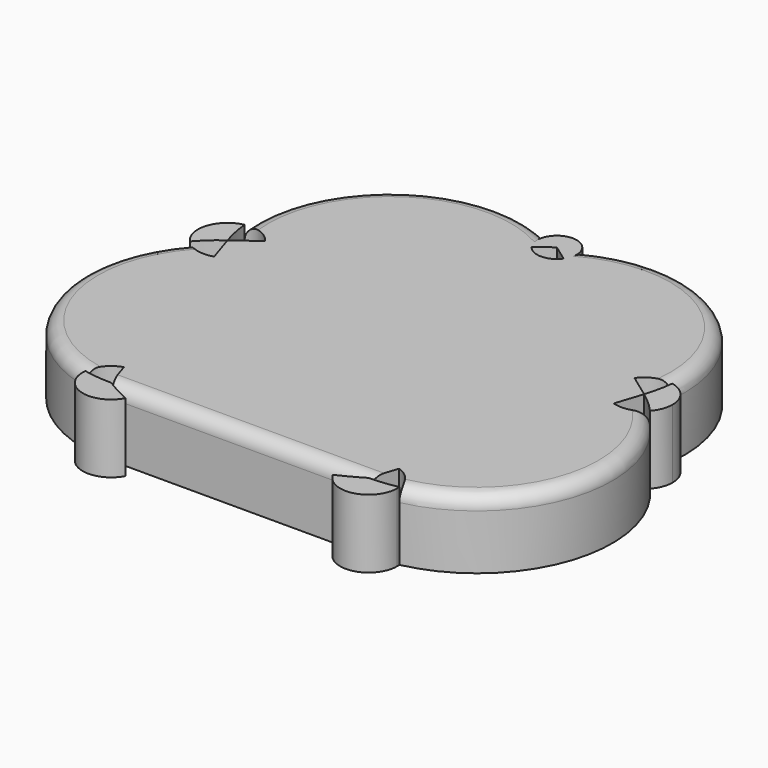
from build123d import *

# Parameters (mm, degrees)
F1_DEPTH     = 25.4
F2_T1_DEPTH  = 105.5253390088
F2_T6_ANGLE  = 135.1802111387
F2_S7_R      = 7.3377134681
F2_T8_DEPTH  = 54
F2_T10_ANGLE = 131.5087282243
F2_T12_ANGLE = 131.0798159324
F2_T16_ANGLE = 134.7112563381
F2_S17_R     = 7.3377134681
F2_T18_DEPTH = 54


# Not quite as in the source:
# - a fillet or chamfer that OpenCascade refuses, or shapes differently, is made with other operations: its cross-section is extruded or revolved along the edge and cut away or added


with BuildPart() as f1:
    # F0 (on Top) → F1 (new body)
    with BuildSketch(Plane.XY):
        with BuildLine():
            ThreePointArc((6.2360330355, 84.9896339964), (0, 88.4603161847), (-6.2360330355, 84.9896339964))
            ThreePointArc((-6.2360330355, 84.9896339964), (-3.047176806, 83.1703555454), (0, 81.1226027166))
            ThreePointArc((0, 81.1226027166), (3.047176806, 83.1703555454), (6.2360330355, 84.9896339964))
        make_face()
        with BuildLine():
            ThreePointArc((-58.1271279807, -64.5296013791), (-55.8437372027, -59.0194503726), (-50.9280340543, -55.6413591785))
            Line((-50.9280340543, -55.6413591785), (-73.7747197353, 14.6735092211))
            ThreePointArc((-73.7747197353, 14.6735092211), (-79.9572494224, 14.504659036), (-85.2415562442, 17.7184239823))
            ThreePointArc((-85.2415562442, 17.7184239823), (-95.2984726264, -31.1903792148), (-58.1271279807, -64.5296013791))
        make_face()
        with BuildLine():
            ThreePointArc((-6.2360330355, 84.9896339964), (-57.4611379356, 82.1562530019), (-79.3764959392, 35.7692235276))
            ThreePointArc((-79.3764959392, 35.7692235276), (-73.2123982771, 35.2631763666), (-68.3098743407, 31.4925739254))
            Line((-68.3098743407, 31.4925739254), (-5.9363348955, 76.8096029546))
            ThreePointArc((-5.9363348955, 76.8096029546), (-7.3327936166, 80.8539454711), (-6.2360330355, 84.9896339964))
        make_face()
        with BuildLine():
            ThreePointArc((0, 81.1226027166), (-3.047176806, 83.1703555454), (-6.2360330355, 84.9896339964))
            ThreePointArc((-6.2360330355, 84.9896339964), (-7.3327936166, 80.8539454711), (-5.9363348955, 76.8096029546))
            Line((-5.9363348955, 76.8096029546), (0, 81.1226027166))
        make_face()
        with BuildLine():
            Line((0, 81.1226027166), (5.9363348955, 76.8096029546))
            ThreePointArc((5.9363348955, 76.8096029546), (6.9785802085, 78.8551245551), (7.3377134681, 81.1226027166))
            ThreePointArc((7.3377134681, 81.1226027166), (7.0569208063, 83.1330523364), (6.2360330355, 84.9896339964))
            ThreePointArc((6.2360330355, 84.9896339964), (3.047176806, 83.1703555454), (0, 81.1226027166))
        make_face()
        with BuildLine():
            Line((5.9363348955, 76.8096029546), (68.6399088663, 31.2527898068))
            ThreePointArc((68.6399088663, 31.2527898068), (73.3795359036, 34.8903954871), (79.3356085511, 35.3609676448))
            ThreePointArc((79.3356085511, 35.3609676448), (57.631102228, 82.041368379), (6.2360330355, 84.9896339964))
            ThreePointArc((6.2360330355, 84.9896339964), (7.0569208063, 83.1330523364), (7.3377134681, 81.1226027166))
            ThreePointArc((7.3377134681, 81.1226027166), (6.9785802085, 78.8551245551), (5.9363348955, 76.8096029546))
        make_face()
        with BuildLine():
            Line((73.9007817067, 15.061488075), (50.9387999635, -55.6082251168))
            ThreePointArc((50.9387999635, -55.6082251168), (55.8696514193, -58.9960922671), (58.1613893706, -64.5222914193))
            ThreePointArc((58.1613893706, -64.5222914193), (95.3677177171, -30.9787541574), (84.9685108653, 18.0246769258))
            ThreePointArc((84.9685108653, 18.0246769258), (79.8733514993, 14.9044861347), (73.9007817067, 15.061488075))
        make_face()
        with BuildLine():
            ThreePointArc((-50.9280340543, -55.6413591785), (-41.5096192986, -57.1330895283), (-37.1804492093, -65.6295642257))
            Line((-37.1804492093, -65.6295642257), (37.1456099952, -65.6295642257))
            ThreePointArc((37.1456099952, -65.6295642257), (41.4891413224, -57.104904012), (50.9387999635, -55.6082251168))
            Line((50.9387999635, -55.6082251168), (73.9007817067, 15.061488075))
            ThreePointArc((73.9007817067, 15.061488075), (67.1454051401, 21.8168646416), (68.6399088663, 31.2527898068))
            Line((68.6399088663, 31.2527898068), (5.9363348955, 76.8096029546))
            ThreePointArc((5.9363348955, 76.8096029546), (0, 73.7848892486), (-5.9363348955, 76.8096029546))
            Line((-5.9363348955, 76.8096029546), (-68.3098743407, 31.4925739254))
            ThreePointArc((-68.3098743407, 31.4925739254), (-66.7574262862, 28.4457230645), (-66.2224891432, 25.0682628674))
            ThreePointArc((-66.2224891432, 25.0682628674), (-68.3098743407, 18.6439518093), (-73.7747197353, 14.6735092211))
            Line((-73.7747197353, 14.6735092211), (-50.9280340543, -55.6413591785))
        make_face()
        with BuildLine():
            ThreePointArc((68.6399088663, 31.2527898068), (67.1454051401, 21.8168646416), (73.9007817067, 15.061488075))
            Line((73.9007817067, 15.061488075), (77.1521799325, 25.0682628674))
            Line((77.1521799325, 25.0682628674), (68.6399088663, 31.2527898068))
        make_face()
        with BuildLine():
            Line((-77.1521799325, 25.0682628674), (-73.7747197353, 14.6735092211))
            ThreePointArc((-73.7747197353, 14.6735092211), (-68.3098743407, 18.6439518093), (-66.2224891432, 25.0682628674))
            ThreePointArc((-66.2224891432, 25.0682628674), (-66.7574262862, 28.4457230645), (-68.3098743407, 31.4925739254))
            Line((-68.3098743407, 31.4925739254), (-77.1521799325, 25.0682628674))
        make_face()
        with BuildLine():
            ThreePointArc((50.9387999635, -55.6082251168), (41.4891413224, -57.104904012), (37.1456099952, -65.6295642257))
            Line((37.1456099952, -65.6295642257), (47.6826695044, -65.6295642257))
            Line((47.6826695044, -65.6295642257), (50.9387999635, -55.6082251168))
        make_face()
        with BuildLine():
            Line((-47.6826695044, -65.6295642257), (-37.1804492093, -65.6295642257))
            ThreePointArc((-37.1804492093, -65.6295642257), (-41.5096192986, -57.1330895283), (-50.9280340543, -55.6413591785))
            Line((-50.9280340543, -55.6413591785), (-47.6826695044, -65.6295642257))
        make_face()
    extrude(amount=F1_DEPTH)

    # F2: fillet of radius 5.08 on 5 edges, made by hand

    # F2_s2 → F2_t1 (cut)
    with BuildSketch(Plane.YZ.offset(-52.7626695044)):
        with BuildLine():
            ThreePointArc((-65.6295642257, 20.32), (-64.1416666741, 23.9121024484), (-60.5495642257, 25.4))
            Line((-60.5495642257, 25.4), (-60.5495642257, 25.5016))
            Line((-60.5495642257, 25.5016), (-65.7311642257, 25.5016))
            Line((-65.7311642257, 25.5016), (-65.7311642257, 20.32))
            Line((-65.7311642257, 20.32), (-65.6295642257, 20.32))
        make_face()
    extrude(amount=F2_T1_DEPTH, mode=Mode.SUBTRACT)


with BuildPart() as f1b:
    # F0 (on Top) → F1, piece 2 (new body)
    with BuildSketch(Plane.XY):
        with BuildLine():
            ThreePointArc((77.1521799325, 25.0682628674), (81.2456293537, 21.7520811746), (84.9685108653, 18.0246769258))
            ThreePointArc((84.9685108653, 18.0246769258), (86.9743125522, 21.2956188385), (87.6739256131, 25.0682628674))
            ThreePointArc((87.6739256131, 25.0682628674), (85.3277720457, 31.6914664552), (79.3356085511, 35.3609676448))
            ThreePointArc((79.3356085511, 35.3609676448), (78.514647387, 30.157179414), (77.1521799325, 25.0682628674))
        make_face()
    extrude(amount=F1_DEPTH)


with BuildPart() as f1c:
    # F0 (on Top) → F1, piece 3 (new body)
    with BuildSketch(Plane.XY):
        with BuildLine():
            ThreePointArc((58.1613893706, -64.5222914193), (52.951199259, -65.3519775789), (47.6826695044, -65.6295642257))
            ThreePointArc((47.6826695044, -65.6295642257), (43.1052780453, -68.2425867862), (38.3851745007, -70.5880125472))
            ThreePointArc((38.3851745007, -70.5880125472), (50.2381895063, -75.8520365597), (58.2197290136, -65.6295642257))
            ThreePointArc((58.2197290136, -65.6295642257), (58.205133995, -65.0751599099), (58.1613893706, -64.5222914193))
        make_face()
    extrude(amount=F1_DEPTH)


with BuildPart() as f1d:
    # F0 (on Top) → F1, piece 4 (new body)
    with BuildSketch(Plane.XY):
        with BuildLine():
            ThreePointArc((-38.4168568148, -70.573383228), (-43.1206730546, -68.2343745884), (-47.6826695044, -65.6295642257))
            ThreePointArc((-47.6826695044, -65.6295642257), (-52.933779652, -65.3538152094), (-58.1271279807, -64.5296013791))
            ThreePointArc((-58.1271279807, -64.5296013791), (-50.7614884715, -75.6703562709), (-38.4168568148, -70.573383228))
        make_face()
    extrude(amount=F1_DEPTH)


with BuildPart() as f1e:
    # F0 (on Top) → F1, piece 5 (new body)
    with BuildSketch(Plane.XY):
        with BuildLine():
            ThreePointArc((-79.3764959392, 35.7692235276), (-87.5469335787, 28.4457230645), (-85.2415562442, 17.7184239823))
            ThreePointArc((-85.2415562442, 17.7184239823), (-81.3977483213, 21.614436135), (-77.1521799325, 25.0682628674))
            ThreePointArc((-77.1521799325, 25.0682628674), (-78.5568084926, 30.357949876), (-79.3764959392, 35.7692235276))
        make_face()
    extrude(amount=F1_DEPTH)


with BuildPart() as f2_tool4:
    # F2_s5 → F2_t6 (revolve)
    with BuildSketch(Plane(origin=(9.3204559106, 44.7572347186, 0), x_dir=(0, 0, 1), z_dir=(-0.2038710699, -0.9789977461, 0))):
        with BuildLine():
            ThreePointArc((20.32, -70.7178341167), (23.9121024484, -69.2299365651), (25.4, -65.6378341167))
            Line((25.4, -65.6378341167), (25.5016, -65.6378341167))
            Line((25.5016, -65.6378341167), (25.5016, -70.8194341167))
            Line((25.5016, -70.8194341167), (20.32, -70.8194341167))
            Line((20.32, -70.8194341167), (20.32, -70.7178341167))
        make_face()
    revolve(axis=Axis((29.4695104281, 40.5613013583, 25.4), (0, 0, 1)), revolution_arc=F2_T6_ANGLE)

    # F2_s7 → F2_t8 (cut, symmetric)
    with BuildSketch(Plane.XY.offset(22.9)):
        with Locations((0, 81.1226027166)):
            Circle(F2_S7_R)
    extrude(amount=F2_T8_DEPTH, both=True, mode=Mode.SUBTRACT)


with BuildPart() as f1_1:
    add(f1.part)

    # F2_t3: cut F2_tool4
    add(f2_tool4.part, mode=Mode.SUBTRACT)

    # F2_s9 → F2_t10 (revolve, cut)
    with BuildSketch(Plane(origin=(45.4389111896, 4.9799294037, 0), x_dir=(0, 0, 1), z_dir=(-0.9940479087, -0.1089438166, 0))):
        with BuildLine():
            ThreePointArc((20.32, -70.73208025), (23.9121024484, -69.2441826984), (25.4, -65.65208025))
            Line((25.4, -65.65208025), (25.5016, -65.65208025))
            Line((25.5016, -65.65208025), (25.5016, -70.83368025))
            Line((25.5016, -70.83368025), (20.32, -70.83368025))
            Line((20.32, -70.83368025), (20.32, -70.73208025))
        make_face()
    revolve(axis=Axis((47.6826695044, -15.4930384909, 25.4), (0, 0, 1)), revolution_arc=F2_T10_ANGLE, mode=Mode.SUBTRACT)

    # F2_s11 → F2_t12 (revolve, cut)
    with BuildSketch(Plane(origin=(-33.4703017863, -30.8917303494, 0), x_dir=(0, 0, 1), z_dir=(0.7348464783, 0.67823348, 0))):
        with BuildLine():
            ThreePointArc((20.32, -71.0915038331), (23.9121024484, -69.6036062816), (25.4, -66.0115038331))
            Line((25.4, -66.0115038331), (25.5016, -66.0115038331))
            Line((25.5016, -66.0115038331), (25.5016, -71.1931038331))
            Line((25.5016, -71.1931038331), (20.32, -71.1931038331))
            Line((20.32, -71.1931038331), (20.32, -71.0915038331))
        make_face()
    revolve(axis=Axis((-47.6826695044, -15.4930384909, 25.4), (0, 0, 1)), revolution_arc=F2_T12_ANGLE, mode=Mode.SUBTRACT)


with BuildPart() as f2_tool14:
    # F2_s15 → F2_t16 (revolve)
    with BuildSketch(Plane(origin=(-39.1768027241, 25.8487847204, 0), x_dir=(0, 0, 1), z_dir=(0.8346868287, -0.5507248842, 0))):
        with BuildLine():
            ThreePointArc((20.32, -67.7629170143), (23.9121024484, -66.2750194628), (25.4, -62.6829170143))
            Line((25.4, -62.6829170143), (25.5016, -62.6829170143))
            Line((25.5016, -62.6829170143), (25.5016, -67.8645170143))
            Line((25.5016, -67.8645170143), (20.32, -67.8645170143))
            Line((20.32, -67.8645170143), (20.32, -67.7629170143))
        make_face()
    revolve(axis=Axis((-29.4695104281, 40.5613013583, 25.4), (0, 0, 1)), revolution_arc=F2_T16_ANGLE)

    # F2_s17 → F2_t18 (cut, symmetric)
    with BuildSketch(Plane.XY.offset(22.9)):
        with Locations((0, 81.1226027166)):
            Circle(F2_S17_R)
    extrude(amount=F2_T18_DEPTH, both=True, mode=Mode.SUBTRACT)


with BuildPart() as f1_2:
    add(f1_1.part)

    # F2_t13: cut F2_tool14
    add(f2_tool14.part, mode=Mode.SUBTRACT)


solid = Compound([f1b.part, f1c.part, f1d.part, f1e.part, f1_2.part])
